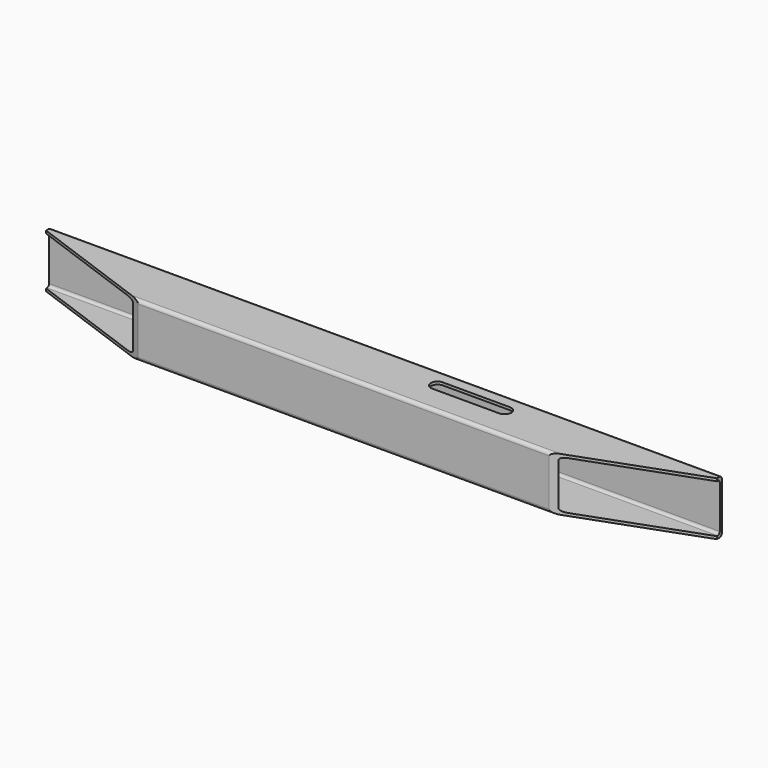
from build123d import *

# Parameters (mm, degrees)
F1_DEPTH = 500
F3_DEPTH = 80
F5_DEPTH = 80.001


# Not quite as in the source:
# - a pattern or mirror of a feature is missing from the dataset's text; its kind, count and spacing are read off the source's solid


with BuildPart() as f1:
    # F0 (on Right) → F1 (new body, symmetric)
    with BuildSketch(Plane.YZ):
        with BuildLine():
            Line((35, 40), (-35, 40))
            ThreePointArc((-35, 40), (-38.5355339059, 38.5355339059), (-40, 35))
            Line((-40, 35), (-40, -35))
            ThreePointArc((-40, -35), (-38.5355339059, -38.5355339059), (-35, -40))
            Line((-35, -40), (35, -40))
            ThreePointArc((35, -40), (38.5355339059, -38.5355339059), (40, -35))
            Line((40, -35), (40, 35))
            ThreePointArc((40, 35), (38.5355339059, 38.5355339059), (35, 40))
        make_face()
        with BuildLine():
            ThreePointArc((-36, 32), (-34.8284271247, 34.8284271247), (-32, 36))
            Line((-32, 36), (32, 36))
            ThreePointArc((32, 36), (34.8284271247, 34.8284271247), (36, 32))
            Line((36, 32), (36, -32))
            ThreePointArc((36, -32), (34.8284271247, -34.8284271247), (32, -36))
            Line((32, -36), (-32, -36))
            ThreePointArc((-32, -36), (-34.8284271247, -34.8284271247), (-36, -32))
            Line((-36, -32), (-36, 32))
        make_face(mode=Mode.SUBTRACT)
    extrude(amount=F1_DEPTH, both=True)

    # F2 (on face) → F3 (cut, through all)
    with BuildSketch(Plane.XY.offset(40)):
        Polygon((-500, 30.4411906294), (-540, 45), (-540, -54.9271104923), (-265.4525203311, -54.9271104923), (-320.2018064436, -35), (-500, -35), align=None)
        Polygon((-320.2018064436, -35), (-500, 30.4411906294), (-500, -35), align=None)
    f3 = extrude(amount=-F3_DEPTH, mode=Mode.SUBTRACT)

    # F3_copies: F3 across plane
    add(f3.mirror(Plane(origin=(0, 0, 0), x_dir=(0, 0, 1), z_dir=(1, 0, 0))), mode=Mode.SUBTRACT)

    # F4 (on face) → F5 (cut, through all)
    with BuildSketch(Plane.XY.offset(40)):
        with BuildLine():
            Line((100, 0), (200, 0))
            ThreePointArc((200, 0), (210, 10), (200, 20))
            Line((200, 20), (100, 20))
            ThreePointArc((100, 20), (90, 10), (100, 0))
        make_face()
    extrude(amount=-F5_DEPTH, mode=Mode.SUBTRACT)


solid = f1.part
